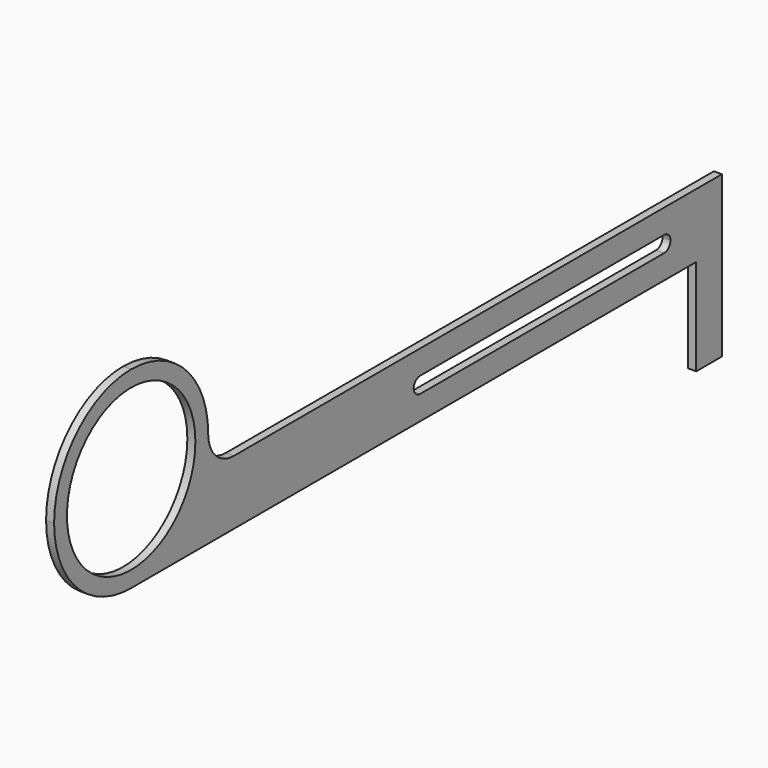
from build123d import *

# Parameters (mm, degrees)
F1_DEPTH = 1.5875
F2_R     = 19.04999
F3_R     = 6.35
F4_R     = 15.875
F5_DEPTH = 25.4
F6_W     = 63.5
F6_H     = 3.175
F7_DEPTH = 25.4
F8_R     = 1.58749


# Not quite as in the source:
# - a fillet or chamfer is up to 0.001 mm smaller than in the source, because OpenCascade refuses the exact size


with BuildPart() as f1:
    # F0 (on Right) → F1 (new body)
    with BuildSketch(Plane.YZ):
        Polygon((-63.1363113923, 43.5325428513), (-101.2363113923, 43.5325428513), (-101.2363113923, 5.4325428513), (57.5136886077, 5.4325428513), (57.5136886077, -13.6174602094), (63.8636886077, -13.6174602094), (63.8636886077, 18.1325428513), (-63.1363113923, 18.1325428513), align=None)
    extrude(amount=F1_DEPTH)

    # F2 (radius 19.05 in the source; OpenCascade refuses exactly that, so slightly less here)
    f2_edges = [f1.edges().sort_by_distance(p)[0] for p in [
        (0.79375, -63.136311, 43.532543),
        (0.79375, -101.236311, 43.532543),
        (0.79375, -101.236311, 5.432543),
    ]]
    fillet(f2_edges, radius=F2_R)

    # F3
    f3_edges = [f1.edges().sort_by_distance(p)[0] for p in [
        (0.79375, -63.136311, 18.132543),
    ]]
    fillet(f3_edges, radius=F3_R)

    # F4 (on face) → F5 (cut)
    with BuildSketch(Plane.YZ.offset(1.5875)):
        with Locations((-82.1863113923, 24.4825428513)):
            Circle(F4_R)
    extrude(amount=-F5_DEPTH, mode=Mode.SUBTRACT)

    # F6 (on face) → F7 (cut)
    with BuildSketch(Plane.YZ.offset(1.5875)):
        with Locations((19.4136886077, 11.7825428513)):
            Rectangle(F6_W, F6_H)
    extrude(amount=-F7_DEPTH, mode=Mode.SUBTRACT)

    # F8 (radius 1.5875 in the source; OpenCascade refuses exactly that, so slightly less here)
    f8_edges = [f1.edges().sort_by_distance(p)[0] for p in [
        (0.79375, -12.336311, 13.370043),
        (0.79375, -12.336311, 10.195043),
        (0.79375, 51.163689, 10.195043),
        (0.79375, 51.163689, 13.370043),
    ]]
    fillet(f8_edges, radius=F8_R)


solid = f1.part
